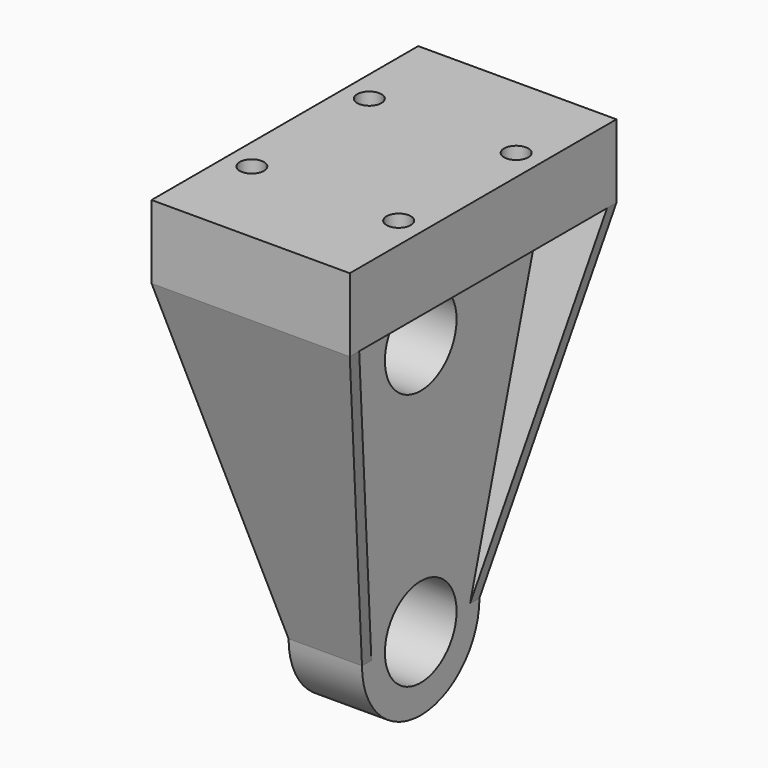
from build123d import *

# Parameters (mm, degrees)
F0_R           = 6.1
F1_DEPTH       = 10
F2_W           = 8.5
F2_H           = 45.4
F2_W_2         = 10
F3_DEPTH       = 10
F5_D           = 3.3
F5_CBORE_D     = 6.5
F5_CBORE_DEPTH = 3
F7_DEPTH       = 8.5
F7_DEPTH_BACK  = 18.5
F9_DEPTH       = 45.401


with BuildPart() as f1:
    # F0 (on Right) → F1 (new body)
    with BuildSketch(Plane.YZ):
        with BuildLine():
            Line((22.7, 0), (0, 0))
            Line((0, 0), (-22.7, 0))
            Line((-22.7, 0), (-10, -45))
            ThreePointArc((-10, -45), (0, -35), (10, -45))
            Line((10, -45), (22.7, 0))
        make_face()
        with Locations((0, -10)):
            Circle(F0_R, mode=Mode.SUBTRACT)
        with BuildLine():
            ThreePointArc((10, -45), (0, -35), (-10, -45))
            ThreePointArc((-10, -45), (0, -55), (10, -45))
        make_face()
        with Locations((0, -45)):
            Circle(F0_R, mode=Mode.SUBTRACT)
    extrude(amount=F1_DEPTH)

    # F2 (on face) → F3 (join)
    with BuildSketch(Plane.XY):
        with Locations((14.25, 0)):
            Rectangle(F2_W, F2_H)
        with Locations((5, 0)):
            Rectangle(F2_W_2, F2_H)
        with Locations((-4.25, 0)):
            Rectangle(F2_W, F2_H)
    extrude(amount=F3_DEPTH)

    # F5 (through all)
    with Locations(Plane(origin=(0, 0, 0), x_dir=(1, 0, 0), z_dir=(0, 0, -1))):
        with Locations((-5, 10), (15, 10), (15, -10), (-5, -10)):
            CounterBoreHole(F5_D / 2, F5_CBORE_D / 2, F5_CBORE_DEPTH)

    # F6 (on face) → F7 (join, two sides)
    with BuildSketch(Plane.YZ.offset(10)) as f7_sk:
        with BuildLine():
            Line((21.1, 0), (8.4, -45))
            ThreePointArc((8.4, -45), (0, -53.4), (-8.4, -45))
            Line((-8.4, -45), (-21.1, 0))
            Line((-21.1, 0), (-22.7, 0))
            Line((-22.7, 0), (-10, -45))
            ThreePointArc((-10, -45), (0, -55), (10, -45))
            Line((10, -45), (22.7, 0))
            Line((22.7, 0), (21.1, 0))
        make_face()
    extrude(amount=F7_DEPTH)
    extrude(f7_sk.sketch, amount=-F7_DEPTH_BACK)

    # F8 (on face) → F9 (cut, through all)
    with BuildSketch(Plane.XZ.offset(22.7)):
        Polygon((0, -45), (-8.5, 0), (-8.5, -58.9339546859), (18.5, -58.9339546859), (18.5, 0), (10, -45), (10, -55), (0, -55), align=None)
    extrude(amount=-F9_DEPTH, mode=Mode.SUBTRACT)


solid = f1.part
